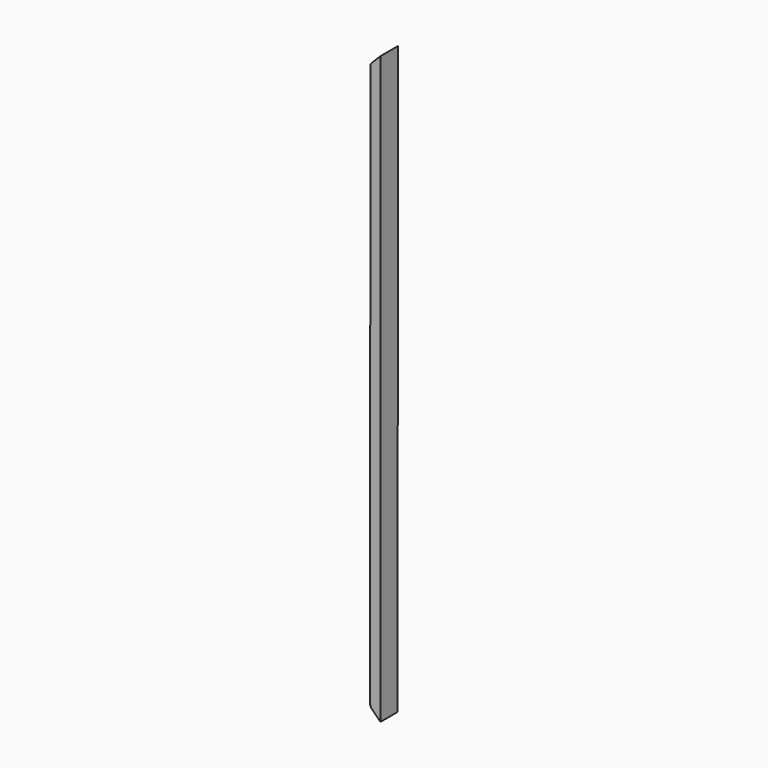
from build123d import *

# Parameters (mm, degrees)
F1_DEPTH = 18


# Not quite as in the source:
# - ends of sketch curves that miss each other by under 0.0002 mm in the source are joined


with BuildPart() as f1:
    # F0 (on Front) → F1 (new body)
    with BuildSketch(Plane.XZ):
        with BuildLine():
            ThreePointArc((-10.2488967252, -146.3380451174), (-9.9448538694, -147.8688662998), (-9.0781349308, -149.1668084527))
            Line((-9.0781349308, -149.1668084527), (-1.6450976958, -156.604110485))
            Line((-1.6450976958, -156.604110485), (-1.5045689609, 333.3958698635))
            Line((-1.5045689609, 333.3958698635), (-8.9418702467, 325.9628326518))
            ThreePointArc((-8.9418702467, 325.9628326518), (-9.8093334866, 324.6653878578), (-10.1142545458, 323.1347414317))
            Line((-10.1142545458, 323.1347414317), (-10.2488967252, -146.3380451174))
        make_face()
    extrude(amount=F1_DEPTH)


solid = f1.part
